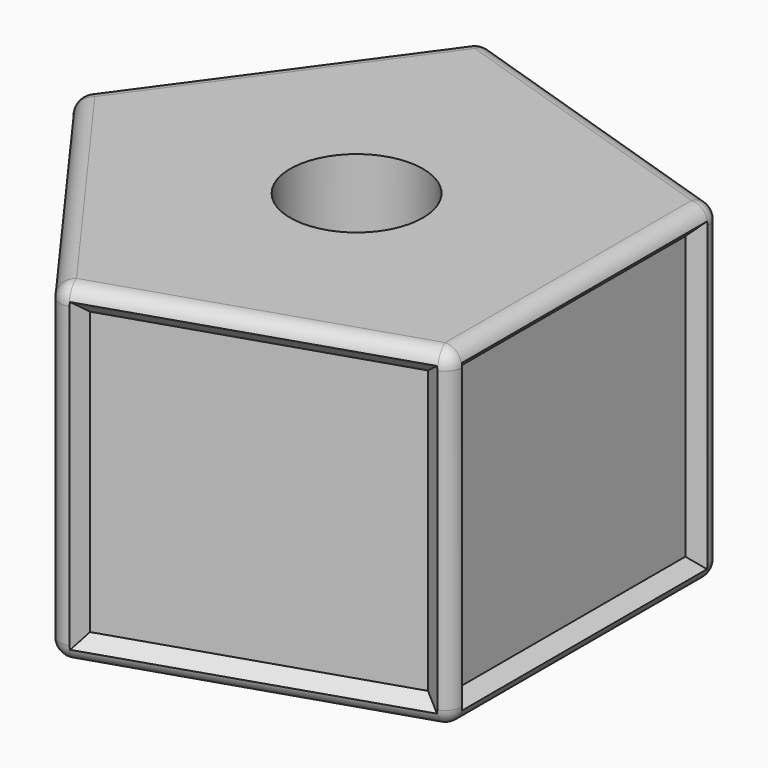
from build123d import *

# Parameters (mm, degrees)
F0_R            = 8
F1_DEPTH        = 40
F2_W            = 37
F2_H            = 37
F3_DEPTH        = 1.5
F3_COPIES_COUNT = 5
F4_SIZE         = 1.49999
F5_R            = 3
F6_DEPTH        = 20
F7_R            = 2
F8_T1_DEPTH     = 37.093829888
F8_T3_DEPTH     = 37.093829888
F8_T5_DEPTH     = 37.093829888
F8_T7_DEPTH     = 37.093829888
F8_T9_DEPTH     = 37.093829888
F8_T12_ANGLE    = 72
F8_T14_ANGLE    = 72
F8_T16_ANGLE    = 72
F8_T18_ANGLE    = 72
F8_T20_ANGLE    = 72
F8_T22_ANGLE    = 72
F8_T24_ANGLE    = 72
F8_T26_ANGLE    = 72
F8_T28_ANGLE    = 72
F8_T30_ANGLE    = 72
F9_R            = 1.5
F10_DEPTH       = 10


# Not quite as in the source:
# - a fillet or chamfer that OpenCascade refuses, or shapes differently, is made with other operations: its cross-section is extruded or revolved along the edge and cut away or added
# - a fillet or chamfer is up to 0.001 mm smaller than in the source, because OpenCascade refuses the exact size
# - a pattern or mirror of a feature is missing from the dataset's text; its kind, count and spacing are read off the source's solid


with BuildPart() as f1:
    # F0 (on Top) → F1 (new body)
    with BuildSketch(Plane.XY):
        Polygon((27.5276384094, -20), (27.5276384094, 20), (-10.5146222424, 32.360679775), (-34.0260323341, 0), (-10.5146222424, -32.360679775), align=None)
        Circle(F0_R, mode=Mode.SUBTRACT)
    extrude(amount=F1_DEPTH)

    # F2 (on face) → F3 (cut)
    with BuildSketch(Plane.YZ.offset(27.5276384094)):
        with Locations((0, 20)):
            Rectangle(F2_W, F2_H)
    f3 = extrude(amount=-F3_DEPTH, mode=Mode.SUBTRACT)

    # F3_copies: F3 ×5 about axis
    f3_copies_axis = Axis((0, 0, 0), (0, 0, 1))
    for i in range(1, F3_COPIES_COUNT):
        add(f3.rotate(f3_copies_axis, i * 360 / F3_COPIES_COUNT), mode=Mode.SUBTRACT)

    # F4 (size 1.5 in the source; OpenCascade refuses exactly that, so slightly less here)
    f4_edges = [f1.edges().sort_by_distance(p)[0] for p in [
        (26.027638, 0, 38.5),
        (26.027638, -18.5, 20),
        (26.027638, 0, 1.5),
        (26.027638, 18.5, 20),
        (25.637528, -19.036941, 20),
        (8.042983, -24.753755, 1.5),
        (-9.551563, -30.47057, 20),
        (8.042983, -24.753755, 38.5),
        (-9.551563, 30.47057, 20),
        (8.042983, 24.753755, 1.5),
        (25.637528, 19.036941, 20),
        (8.042983, 24.753755, 38.5),
        (-10.182775, -30.265476, 20),
        (-21.056802, -15.298662, 1.5),
        (-31.930829, -0.331848, 20),
        (-21.056802, -15.298662, 38.5),
        (-31.930829, 0.331848, 20),
        (-21.056802, 15.298662, 1.5),
        (-10.182775, 30.265476, 20),
        (-21.056802, 15.298662, 38.5),
    ]]
    chamfer(f4_edges, length=F4_SIZE)

    # F5 (on Right) → F6 (cut)
    with BuildSketch(Plane.YZ):
        with Locations((0, 49.5)):
            Circle(F5_R)
    extrude(amount=F6_DEPTH, mode=Mode.SUBTRACT)

    # F7
    f7_edges = [f1.edges().sort_by_distance(p)[0] for p in [
        (-34.026032, 0, 20),
        (-10.514622, -32.36068, 20),
        (27.527638, -20, 20),
        (27.527638, 20, 20),
        (-10.514622, 32.36068, 20),
    ]]
    fillet(f7_edges, radius=F7_R)

    # F8: fillet of radius 2 on 12 edges, made by hand

    # F8_s2 → F8_t1 (cut)
    with BuildSketch(Plane(origin=(-17.6391643147, -5.7313119109, 0), x_dir=(0, 0, 1), z_dir=(0.9510565163, 0.3090169944, 0))):
        with BuildLine():
            ThreePointArc((40, 25.5276384094), (39.4142135624, 26.9418519718), (38, 27.5276384094))
            Line((38, 27.5276384094), (40, 27.5276384094))
            Line((40, 27.5276384094), (40, 25.5276384094))
        make_face()
        with BuildLine():
            ThreePointArc((0, 25.5276384094), (0.5857864376, 26.9418519718), (2, 27.5276384094))
            Line((2, 27.5276384094), (0, 27.5276384094))
            Line((0, 27.5276384094), (0, 25.5276384094))
        make_face()
    extrude(amount=F8_T1_DEPTH, mode=Mode.SUBTRACT)

    # F8_s4 → F8_t3 (cut)
    with BuildSketch(Plane(origin=(-10.9016030796, 15.0047693829, 0), x_dir=(0, 0, 1), z_dir=(0.5877852523, -0.8090169944, 0))):
        with BuildLine():
            ThreePointArc((40, 25.5276384094), (39.4142135624, 26.9418519718), (38, 27.5276384094))
            Line((38, 27.5276384094), (40, 27.5276384094))
            Line((40, 27.5276384094), (40, 25.5276384094))
        make_face()
        with BuildLine():
            ThreePointArc((0, 25.5276384094), (0.5857864376, 26.9418519718), (2, 27.5276384094))
            Line((2, 27.5276384094), (0, 27.5276384094))
            Line((0, 27.5276384094), (0, 25.5276384094))
        make_face()
    extrude(amount=F8_T3_DEPTH, mode=Mode.SUBTRACT)

    # F8_s6 → F8_t5 (cut)
    with BuildSketch(Plane(origin=(10.9016030796, 15.0047693829, 0), x_dir=(0, 0, 1), z_dir=(-0.5877852523, -0.8090169944, 0))):
        with BuildLine():
            ThreePointArc((40, 25.5276384094), (39.4142135624, 26.9418519718), (38, 27.5276384094))
            Line((38, 27.5276384094), (40, 27.5276384094))
            Line((40, 27.5276384094), (40, 25.5276384094))
        make_face()
        with BuildLine():
            ThreePointArc((0, 25.5276384094), (0.5857864376, 26.9418519718), (2, 27.5276384094))
            Line((2, 27.5276384094), (0, 27.5276384094))
            Line((0, 27.5276384094), (0, 25.5276384094))
        make_face()
    extrude(amount=F8_T5_DEPTH, mode=Mode.SUBTRACT)

    # F8_s8 → F8_t7 (cut)
    with BuildSketch(Plane(origin=(17.6391643147, -5.7313119109, 0), x_dir=(0, 0, 1), z_dir=(-0.9510565163, 0.3090169944, 0))):
        with BuildLine():
            ThreePointArc((40, 25.5276384094), (39.4142135624, 26.9418519718), (38, 27.5276384094))
            Line((38, 27.5276384094), (40, 27.5276384094))
            Line((40, 27.5276384094), (40, 25.5276384094))
        make_face()
        with BuildLine():
            ThreePointArc((0, 25.5276384094), (0.5857864376, 26.9418519718), (2, 27.5276384094))
            Line((2, 27.5276384094), (0, 27.5276384094))
            Line((0, 27.5276384094), (0, 25.5276384094))
        make_face()
    extrude(amount=F8_T7_DEPTH, mode=Mode.SUBTRACT)

    # F8_s10 → F8_t9 (cut)
    with BuildSketch(Plane.XZ.offset(-18.546914944)):
        with BuildLine():
            ThreePointArc((27.5276384094, 38), (26.9418519718, 39.4142135624), (25.5276384094, 40))
            Line((25.5276384094, 40), (27.5276384094, 40))
            Line((27.5276384094, 40), (27.5276384094, 38))
        make_face()
        with BuildLine():
            ThreePointArc((27.5276384094, 2), (26.9418519718, 0.5857864376), (25.5276384094, 0))
            Line((25.5276384094, 0), (27.5276384094, 0))
            Line((27.5276384094, 0), (27.5276384094, 2))
        make_face()
    extrude(amount=F8_T9_DEPTH, mode=Mode.SUBTRACT)

    # F8_s11 → F8_t12 (revolve, cut)
    with BuildSketch(Plane.XZ.offset(18.546914944)):
        with BuildLine():
            ThreePointArc((25.5276384094, 0), (26.9418519718, 0.5857864376), (27.5276384094, 2))
            Line((27.5276384094, 2), (27.5276384094, 0))
            Line((27.5276384094, 0), (25.5276384094, 0))
        make_face()
    revolve(axis=Axis((25.5276384094, -18.546914944, 0), (0, 0, -1)), revolution_arc=F8_T12_ANGLE, mode=Mode.SUBTRACT)

    # F8_s13 → F8_t14 (revolve, cut)
    with BuildSketch(Plane.XZ.offset(-18.546914944)):
        with BuildLine():
            ThreePointArc((25.5276384094, 0), (26.9418519718, 0.5857864376), (27.5276384094, 2))
            Line((27.5276384094, 2), (27.5276384094, 0))
            Line((27.5276384094, 0), (25.5276384094, 0))
        make_face()
    revolve(axis=Axis((25.5276384094, 18.546914944, 0), (0, 0, 1)), revolution_arc=F8_T14_ANGLE, mode=Mode.SUBTRACT)

    # F8_s15 → F8_t16 (revolve, cut)
    with BuildSketch(Plane(origin=(-17.6391643147, -5.7313119109, 0), x_dir=(0, 0, 1), z_dir=(0.9510565163, 0.3090169944, 0))):
        with BuildLine():
            ThreePointArc((0, 25.5276384094), (0.5857864376, 26.9418519718), (2, 27.5276384094))
            Line((2, 27.5276384094), (0, 27.5276384094))
            Line((0, 27.5276384094), (0, 25.5276384094))
        make_face()
    revolve(axis=Axis((-9.7506902199, -30.0095387658, 0), (0, 0, -1)), revolution_arc=F8_T16_ANGLE, mode=Mode.SUBTRACT)

    # F8_s17 → F8_t18 (revolve, cut)
    with BuildSketch(Plane(origin=(-17.6391643147, 5.7313119109, 0), x_dir=(0, 0, 1), z_dir=(0.9510565163, -0.3090169944, 0))):
        with BuildLine():
            ThreePointArc((0, -25.5276384094), (0.5857864376, -26.9418519718), (2, -27.5276384094))
            Line((2, -27.5276384094), (0, -27.5276384094))
            Line((0, -27.5276384094), (0, -25.5276384094))
        make_face()
    revolve(axis=Axis((-9.7506902199, 30.0095387658, 0), (0, 0, 1)), revolution_arc=F8_T18_ANGLE, mode=Mode.SUBTRACT)

    # F8_s19 → F8_t20 (revolve, cut)
    with BuildSketch(Plane(origin=(-10.9016030796, 15.0047693829, 0), x_dir=(0, 0, 1), z_dir=(0.5877852523, -0.8090169944, 0))):
        with BuildLine():
            ThreePointArc((0, 25.5276384094), (0.5857864376, 26.9418519718), (2, 27.5276384094))
            Line((2, 27.5276384094), (0, 27.5276384094))
            Line((0, 27.5276384094), (0, 25.5276384094))
        make_face()
    revolve(axis=Axis((-31.5538963791, 0, 0), (0, 0, -1)), revolution_arc=F8_T20_ANGLE, mode=Mode.SUBTRACT)

    # F8_s21 → F8_t22 (revolve, cut)
    with BuildSketch(Plane.XZ.offset(18.546914944)):
        with BuildLine():
            ThreePointArc((27.5276384094, 38), (26.9418519718, 39.4142135624), (25.5276384094, 40))
            Line((25.5276384094, 40), (27.5276384094, 40))
            Line((27.5276384094, 40), (27.5276384094, 38))
        make_face()
    revolve(axis=Axis((25.5276384094, -18.546914944, 40), (0, 0, -1)), revolution_arc=F8_T22_ANGLE, mode=Mode.SUBTRACT)

    # F8_s23 → F8_t24 (revolve, cut)
    with BuildSketch(Plane.XZ.offset(-18.546914944)):
        with BuildLine():
            ThreePointArc((27.5276384094, 38), (26.9418519718, 39.4142135624), (25.5276384094, 40))
            Line((25.5276384094, 40), (27.5276384094, 40))
            Line((27.5276384094, 40), (27.5276384094, 38))
        make_face()
    revolve(axis=Axis((25.5276384094, 18.546914944, 40), (0, 0, 1)), revolution_arc=F8_T24_ANGLE, mode=Mode.SUBTRACT)

    # F8_s25 → F8_t26 (revolve, cut)
    with BuildSketch(Plane(origin=(-17.6391643147, -5.7313119109, 0), x_dir=(0, 0, 1), z_dir=(0.9510565163, 0.3090169944, 0))):
        with BuildLine():
            ThreePointArc((40, 25.5276384094), (39.4142135624, 26.9418519718), (38, 27.5276384094))
            Line((38, 27.5276384094), (40, 27.5276384094))
            Line((40, 27.5276384094), (40, 25.5276384094))
        make_face()
    revolve(axis=Axis((-9.7506902199, -30.0095387658, 40), (0, 0, -1)), revolution_arc=F8_T26_ANGLE, mode=Mode.SUBTRACT)

    # F8_s27 → F8_t28 (revolve, cut)
    with BuildSketch(Plane(origin=(-17.6391643147, 5.7313119109, 0), x_dir=(0, 0, 1), z_dir=(0.9510565163, -0.3090169944, 0))):
        with BuildLine():
            ThreePointArc((40, -25.5276384094), (39.4142135624, -26.9418519718), (38, -27.5276384094))
            Line((38, -27.5276384094), (40, -27.5276384094))
            Line((40, -27.5276384094), (40, -25.5276384094))
        make_face()
    revolve(axis=Axis((-9.7506902199, 30.0095387658, 40), (0, 0, 1)), revolution_arc=F8_T28_ANGLE, mode=Mode.SUBTRACT)

    # F8_s29 → F8_t30 (revolve, cut)
    with BuildSketch(Plane(origin=(-10.9016030796, 15.0047693829, 0), x_dir=(0, 0, 1), z_dir=(0.5877852523, -0.8090169944, 0))):
        with BuildLine():
            ThreePointArc((40, 25.5276384094), (39.4142135624, 26.9418519718), (38, 27.5276384094))
            Line((38, 27.5276384094), (40, 27.5276384094))
            Line((40, 27.5276384094), (40, 25.5276384094))
        make_face()
    revolve(axis=Axis((-31.5538963791, 0, 40), (0, 0, -1)), revolution_arc=F8_T30_ANGLE, mode=Mode.SUBTRACT)

    # F9 (on Right) → F10 (cut)
    with BuildSketch(Plane.YZ):
        with Locations((0, 20)):
            Circle(F9_R)
    extrude(amount=F10_DEPTH, mode=Mode.SUBTRACT)


solid = f1.part
